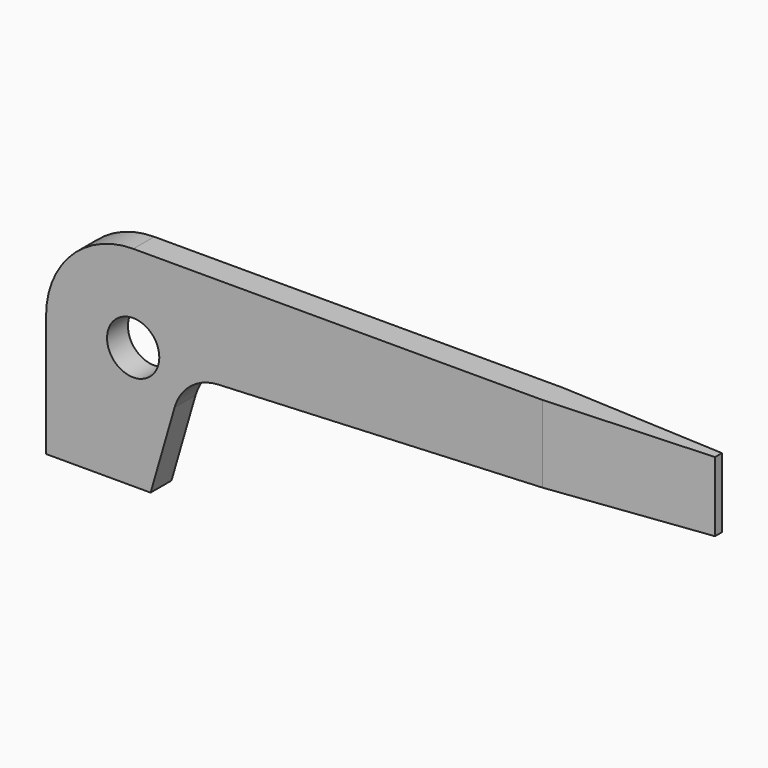
from build123d import *

# Parameters (mm, degrees)
F1_DEPTH = 2.38125
F2_R     = 2.38125
F3_DEPTH = 25.4
F5_DEPTH = 25.4


# Not quite as in the source:
# - a length typed as a fraction of an inch, garbled in the dataset ("3 / 203.2 mm" for 3/8 in), is restored


with BuildPart() as f1:
    # F0 (on Front) → F1 (new body)
    with BuildSketch(Plane.XZ):
        with BuildLine():
            Line((60.325, 19.05), (7.9502, 19.05))
            ThreePointArc((7.9502, 19.05), (2.3285596682, 16.7214403318), (0, 11.0998))
            Line((0, 11.0998), (0, 0))
            Line((0, 0), (9.525, 0))
            Line((9.525, 0), (11.7155767468, 7.5558858532))
            ThreePointArc((11.7155767468, 7.5558858532), (13.1960389642, 9.7526651699), (15.6788970925, 10.6762577523))
            Line((15.6788970925, 10.6762577523), (60.325, 12.7))
            Line((60.325, 12.7), (60.325, 19.05))
        make_face()
    extrude(amount=F1_DEPTH)

    # F2 (on face) → F3 (cut)
    with BuildSketch(Plane.XZ.offset(2.38125)):
        with Locations((7.9375, 11.1125)):
            Circle(F2_R)
    extrude(amount=-F3_DEPTH, mode=Mode.SUBTRACT)

    # F4 (on face) → F5 (cut)
    with BuildSketch(Plane.XY.offset(19.05)):
        Polygon((60.325, 0), (45.24375, 0), (60.325, -0.79375), align=None)
        Polygon((60.325, -2.38125), (60.325, -1.5875), (45.24375, -2.38125), align=None)
    extrude(amount=-F5_DEPTH, mode=Mode.SUBTRACT)


solid = f1.part
